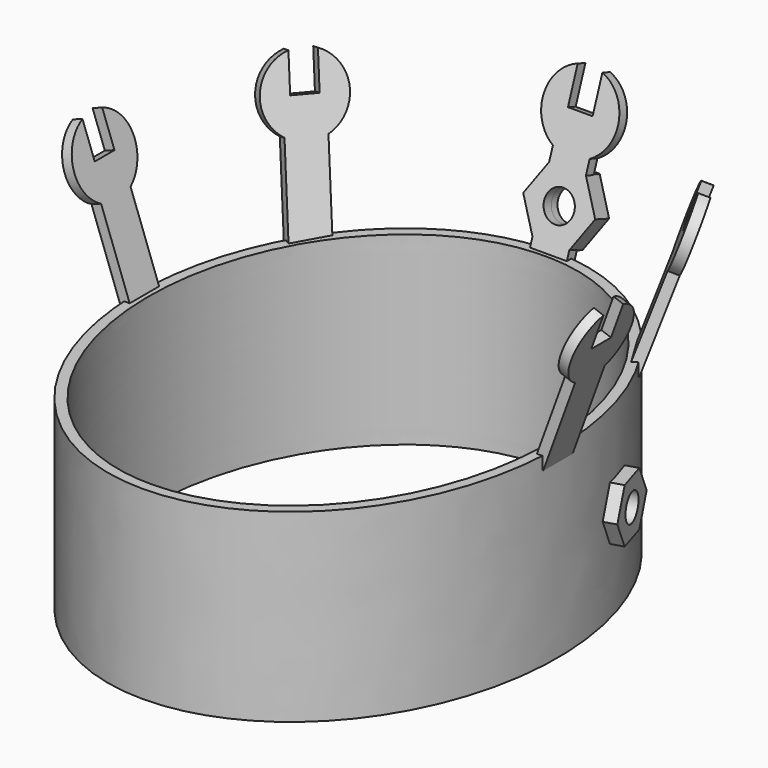
from build123d import *

# Parameters (mm, degrees)
F1_DEPTH       = 45
F6_DEPTH       = 1.25
F6_DEPTH_BACK  = 1.25
F10_COUNT      = 5
F10_ANGLE      = 180
F12_ANGLE      = 15
F14_ANGLE      = -13
F16_R          = 3.6705859031
F17_DEPTH      = 2
F17_DEPTH_BACK = 2.5
F18_DEPTH      = 130.3568903037
F19_R          = 3.3753348164
F20_DEPTH      = 3
F22_ANGLE      = -17.1702382033


# Not quite as in the source:
# - the dataset's text gives a spline's control points without its knots; the knots are read off the source's solid


with BuildPart() as f1:
    # F0 (on Top) → F1 (new body)
    with BuildSketch(Plane.XY):
        with BuildLine():
            add(Edge.make_bspline(
                [(0, -62.5), (88.334591186, -62.5), (44.167295593, 31.25), (0, 125), (-44.167295593, 31.25), (-88.334591186, -62.5), (0, -62.5)],
                knots=[0, 0, 0, 2.0943951024, 2.0943951024, 4.1887902048, 4.1887902048, 6.2831853072, 6.2831853072, 6.2831853072], degree=2, weights=[1, 0.5, 1, 0.5, 1, 0.5, 1]))
        make_face()
        with BuildLine():
            add(Edge.make_bspline(
                [(0, -60), (0.7934400352, -60), (2.3803201055, -59.9516441603), (5.5288309618, -59.664118297), (9.4184732904, -58.9516052433), (13.9818112717, -57.5453727526), (18.4124828933, -55.600757734), (22.6795755459, -53.1302539115), (26.7509819769, -50.1467211333), (29.9537534788, -47.2431908724), (32.3840433605, -44.6780929223), (34.1393054942, -42.6314914397), (35.8116329074, -40.4776143963), (37.9132438089, -37.4874375185), (40.301890819, -33.531442681), (42.768801155, -28.4770439207), (44.8210786115, -23.1549595069), (46.4431748587, -17.6060604033), (47.620169925, -11.8716654292), (48.2179799448, -6.9719744045), (48.459387402, -3.0021151117), (48.520306299, 0), (48.459387402, 3.0021151117), (48.2179799448, 6.9719744045), (47.620169925, 11.8716654292), (46.4431748587, 17.6060604033), (44.8210786115, 23.1549595069), (42.768801155, 28.4770439207), (40.301890819, 33.531442681), (37.9132438089, 37.4874375185), (35.8116329074, 40.4776143963), (34.1393054942, 42.6314914397), (32.3840433605, 44.6780929223), (29.9537534788, 47.2431908724), (26.7509819769, 50.1467211333), (22.6795755459, 53.1302539115), (18.4124828933, 55.600757734), (13.9818112717, 57.5453727526), (9.4184732904, 58.9516052433), (5.5288309618, 59.664118297), (2.3803201055, 59.9516441603), (0, 60.0241779198), (-2.3803201055, 59.9516441603), (-5.5288309618, 59.664118297), (-9.4184732904, 58.9516052433), (-13.9818112717, 57.5453727526), (-18.4124828933, 55.600757734), (-22.6795755459, 53.1302539115), (-26.7509819769, 50.1467211333), (-29.9537534788, 47.2431908724), (-32.3840433605, 44.6780929223), (-34.1393054942, 42.6314914397), (-35.8116329074, 40.4776143963), (-37.9132438089, 37.4874375185), (-40.301890819, 33.531442681), (-42.768801155, 28.4770439207), (-44.8210786115, 23.1549595069), (-46.4431748587, 17.6060604033), (-47.620169925, 11.8716654292), (-48.2179799448, 6.9719744045), (-48.459387402, 3.0021151117), (-48.520306299, 0), (-48.459387402, -3.0021151117), (-48.2179799448, -6.9719744045), (-47.620169925, -11.8716654292), (-46.4431748587, -17.6060604033), (-44.8210786115, -23.1549595069), (-42.768801155, -28.4770439207), (-40.301890819, -33.531442681), (-37.9132438089, -37.4874375185), (-35.8116329074, -40.4776143963), (-34.1393054942, -42.6314914397), (-32.3840433605, -44.6780929223), (-29.9537534788, -47.2431908724), (-26.7509819769, -50.1467211333), (-22.6795755459, -53.1302539115), (-18.4124828933, -55.600757734), (-13.9818112717, -57.5453727526), (-9.4184732904, -58.9516052433), (-5.5288309618, -59.664118297), (-2.3803201055, -59.9516441603), (-0.7934400352, -60), (0, -60)],
                knots=[0, 0, 0, 0, 0.0078125, 0.015625, 0.03125, 0.046875, 0.0625, 0.078125, 0.09375, 0.109375, 0.1171875, 0.125, 0.1328125, 0.140625, 0.15625, 0.171875, 0.1875, 0.203125, 0.21875, 0.234375, 0.2421875, 0.25, 0.2578125, 0.265625, 0.28125, 0.296875, 0.3125, 0.328125, 0.34375, 0.359375, 0.3671875, 0.375, 0.3828125, 0.390625, 0.40625, 0.421875, 0.4375, 0.453125, 0.46875, 0.484375, 0.4921875, 0.5, 0.5078125, 0.515625, 0.53125, 0.546875, 0.5625, 0.578125, 0.59375, 0.609375, 0.6171875, 0.625, 0.6328125, 0.640625, 0.65625, 0.671875, 0.6875, 0.703125, 0.71875, 0.734375, 0.7421875, 0.75, 0.7578125, 0.765625, 0.78125, 0.796875, 0.8125, 0.828125, 0.84375, 0.859375, 0.8671875, 0.875, 0.8828125, 0.890625, 0.90625, 0.921875, 0.9375, 0.953125, 0.96875, 0.984375, 0.9921875, 1, 1, 1, 1], degree=3))
        make_face(mode=Mode.SUBTRACT)
    extrude(amount=F1_DEPTH)


with BuildPart() as f6:
    # F5 (on line) → F6 (new body, two sides)
    with BuildSketch(Plane(origin=(29.4676343046, 0, -10.7253417611), x_dir=(0, 1, 0), z_dir=(0.9396926208, 0, -0.3420201433))) as f6_sk:
        with BuildLine():
            add(Edge.make_bspline(
                [(4.4740695806, 59.6844450689), (0, 59.7740605231), (-4.4740695806, 59.6844450689)],
                knots=[4.6407425869, 4.6407425869, 4.6407425869, 4.7840353739, 4.7840353739, 4.7840353739], degree=2, weights=[1, 0.9974344949, 1]))
            Line((4.4740695806, 59.6844450689), (4.4740695806, 82.335433416))
            ThreePointArc((4.4740695806, 82.335433416), (9.1431267736, 91.1574680805), (3, 99.0245122611))
            Line((3, 99.0245122611), (3, 90.3498977423))
            Line((3, 90.3498977423), (-3, 90.3498977423))
            Line((-3, 90.3498977423), (-3, 99.0245122611))
            ThreePointArc((-3, 99.0245122611), (-9.1431267736, 91.1574680805), (-4.4740695806, 82.335433416))
            Line((-4.4740695806, 82.335433416), (-4.4740695806, 59.6844450689))
        make_face()
    extrude(amount=F6_DEPTH)
    extrude(f6_sk.sketch, amount=-F6_DEPTH_BACK)


with BuildPart() as f6_1:
    # F7: moved
    add(f6.part.moved(Location((0, 0, -3))))


with BuildPart() as f10_1:
    # F10: instance of F6
    add(f6_1.part.rotate(Axis((0, 0, 70.0238226354), (0, 0, 1)), 1 * F10_ANGLE / (F10_COUNT - 1)))


with BuildPart() as f10_2:
    # F10: instance of F6
    add(f6_1.part.rotate(Axis((0, 0, 70.0238226354), (0, 0, 1)), 2 * F10_ANGLE / (F10_COUNT - 1)))


with BuildPart() as f10_3:
    # F10: instance of F6
    add(f6_1.part.rotate(Axis((0, 0, 70.0238226354), (0, 0, 1)), 3 * F10_ANGLE / (F10_COUNT - 1)))


with BuildPart() as f10_4:
    # F10: instance of F6
    add(f6_1.part.rotate(Axis((0, 0, 70.0238226354), (0, 0, 1)), 4 * F10_ANGLE / (F10_COUNT - 1)))


with BuildPart() as f10_2_1:
    # F11: moved
    add(f10_2.part.moved(Location((0, 11.4, 0))))

    # F16 (on face) → F17 (join, two sides)
    with BuildSketch(Plane(origin=(0, 41.6728848209, -15.1676896508), x_dir=(-1, 0, 0), z_dir=(0, 0.9396926208, -0.3420201433))) as f17_sk:
        Polygon((-4.3752939355, 65.1219785213), (4.3752939355, 65.1219785213), (4.4740695806, 65.2930629572), (4.4740695806, 80.1073568741), (4.3752939355, 80.2784413099), (-4.3752939355, 80.2784413099), (-4.4740695806, 80.1073568741), (-4.4740695806, 65.2930629572), align=None)
        with Locations((0, 72.7002099156)):
            Circle(F16_R, mode=Mode.SUBTRACT)
        Polygon((-8.750587871, 72.7002099156), (-4.4740695806, 65.2930629572), (-4.4740695806, 80.1073568741), align=None)
        Polygon((4.4740695806, 80.1073568741), (4.4740695806, 65.2930629572), (8.750587871, 72.7002099156), align=None)
    extrude(amount=F17_DEPTH)
    extrude(f17_sk.sketch, amount=-F17_DEPTH_BACK)

    # F18 (cut, through all): a face of the model
    f18_faces = [f10_2_1.faces().sort_by_distance(p)[0] for p in [
        (0, 66.5378210361, 53.1481611365),
    ]]
    extrude(f18_faces, amount=-F18_DEPTH, mode=Mode.SUBTRACT)


with BuildPart() as f10_3_1:
    # F12: moved
    add(f10_3.part.rotate(Axis((-42.0043696645, 35.6770797846, 52.5746489683), (-0.2418447626, 0.2418447626, 0.9396926208)), F12_ANGLE))


with BuildPart() as f10_3_2:
    # F13: moved
    add(f10_3_1.part.moved(Location((-3.53468, 1.19722, 0))))


with BuildPart() as f10_1_1:
    # F14: moved
    add(f10_1.part.rotate(Axis((40.3432121035, 34.0159222237, 53.4296993266), (0.2418447626, 0.2418447626, 0.9396926208)), F14_ANGLE))


with BuildPart() as f10_1_2:
    # F15: moved
    add(f10_1_1.part.moved(Location((1.71219, 4.34955, 0))))


with BuildPart() as f20:
    # F19 (on offset) → F20 (new body)
    with BuildSketch(Plane.YZ.offset(51)):
        Polygon((19.5871447773, 15.9179512411), (27.1874400228, 15.9179512411), (30.9875876455, 22.5), (27.1874400228, 29.0820487589), (19.5871447773, 29.0820487589), (15.7869971545, 22.5), align=None)
        with Locations((23.3872924, 22.5)):
            Circle(F19_R, mode=Mode.SUBTRACT)
    extrude(amount=F20_DEPTH)


with BuildPart() as f20_1:
    # F22: moved
    add(f20.part.rotate(Axis((51, 19.5871447773, 22.5), (0, 0, -1)), F22_ANGLE))


with BuildPart() as f20_2:
    # F23: moved
    add(f20_1.part.moved(Location((-2.38764, -0.73491, 0))))


solid = Compound([f1.part, f6_1.part, f10_4.part, f10_2_1.part, f10_3_2.part, f10_1_2.part, f20_2.part])
